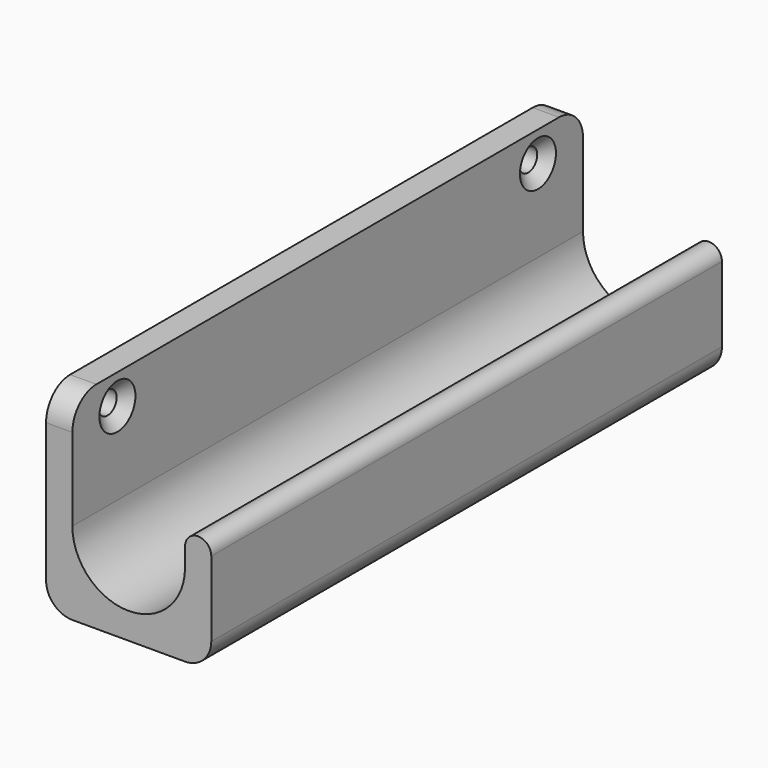
from build123d import *

# Parameters (mm, degrees)
F1_DEPTH  = 107.95
F3_R      = 1.5875
F2_R      = 1.905
F4_DEPTH  = 25.4
F5_SIZE2  = 1.4351924041
F5_SIZE   = 1.651
F7_DEPTH  = 107.95
F8_R      = 1.905
F9_DEPTH  = 25.4
F10_SIZE2 = 1.6559912355
F10_SIZE  = 1.905
F11_R     = 5.08


with BuildPart() as f1:
    # F0 (on Front) → F1 (new body)
    with BuildSketch(Plane.XZ):
        with BuildLine():
            Line((3.175, 0), (0, 0))
            Line((0, 0), (0, -28.575))
            ThreePointArc((0, -28.575), (0.9299359697, -30.8200640303), (3.175, -31.75))
            Line((3.175, -31.75), (22.225, -31.75))
            ThreePointArc((22.225, -31.75), (24.4700640303, -30.8200640303), (25.4, -28.575))
            Line((25.4, -28.575), (25.4, -15.875))
            ThreePointArc((25.4, -15.875), (23.8125, -14.2875), (22.225, -15.875))
            Line((22.225, -15.875), (22.225, -19.05))
            ThreePointArc((22.225, -19.05), (12.7, -28.575), (3.175, -19.05))
            Line((3.175, -19.05), (3.175, 0))
        make_face()
    extrude(amount=F1_DEPTH)

    # F3
    f3_edges = [f1.edges().sort_by_distance(p)[0] for p in [
        (1.5875, 0, 0),
        (1.5875, -107.95, 0),
    ]]
    fillet(f3_edges, radius=F3_R)

    # F2 (on face) → F4 (cut)
    with BuildSketch(Plane(origin=(0, 0, 0), x_dir=(0, -1, 0), z_dir=(-1, 0, 0))):
        with Locations((9.525, -5.08)):
            Circle(F2_R)
        with Locations((98.425, -5.08)):
            Circle(F2_R)
    extrude(amount=-F4_DEPTH, mode=Mode.SUBTRACT)

    # F5
    f5_edges = [f1.edges().sort_by_distance(p)[0] for p in [
        (3.175, -96.52, -5.08),
        (3.175, -7.62, -5.08),
    ]]
    chamfer(f5_edges, length=F5_SIZE, length2=F5_SIZE2)

    # F6 (on face) → F7 (join, through all)
    with BuildSketch(Plane.XZ.offset(107.95)):
        with BuildLine():
            Line((3.175, 0), (0, 0))
            Line((0, 0), (0, -28.575))
            ThreePointArc((0, -28.575), (0.9299359697, -30.8200640303), (3.175, -31.75))
            Line((3.175, -31.75), (22.225, -31.75))
            ThreePointArc((22.225, -31.75), (24.4700640303, -30.8200640303), (25.4, -28.575))
            Line((25.4, -28.575), (25.4, -15.875))
            ThreePointArc((25.4, -15.875), (23.8125, -14.2875), (22.225, -15.875))
            Line((22.225, -15.875), (22.225, -19.05))
            ThreePointArc((22.225, -19.05), (12.7, -28.575), (3.175, -19.05))
            Line((3.175, -19.05), (3.175, 0))
        make_face()
        with BuildLine():
            Line((0, -28.575), (0, 0))
            Line((0, 0), (-1.27, 0))
            Line((-1.27, 0), (-1.27, -28.575))
            ThreePointArc((-1.27, -28.575), (0.0319103576, -31.7180896424), (3.175, -33.02))
            Line((3.175, -33.02), (22.225, -33.02))
            ThreePointArc((22.225, -33.02), (25.3680896424, -31.7180896424), (26.67, -28.575))
            Line((26.67, -28.575), (26.67, -15.875))
            ThreePointArc((26.67, -15.875), (24.4475, -13.6525), (22.225, -15.875))
            ThreePointArc((22.225, -15.875), (23.8125, -14.2875), (25.4, -15.875))
            Line((25.4, -15.875), (25.4, -28.575))
            ThreePointArc((25.4, -28.575), (24.4700640303, -30.8200640303), (22.225, -31.75))
            Line((22.225, -31.75), (3.175, -31.75))
            ThreePointArc((3.175, -31.75), (0.9299359697, -30.8200640303), (0, -28.575))
        make_face()
    extrude(amount=-F7_DEPTH)

    # F8 (on face) → F9 (cut)
    with BuildSketch(Plane(origin=(-1.27, 0, 0), x_dir=(0, -1, 0), z_dir=(-1, 0, 0))):
        with Locations((9.525, -5.08)):
            Circle(F8_R)
        with Locations((98.425, -5.08)):
            Circle(F8_R)
    extrude(amount=-F9_DEPTH, mode=Mode.SUBTRACT)

    # F10
    f10_edges = [f1.edges().sort_by_distance(p)[0] for p in [
        (3.175, -96.52, -5.08),
        (3.175, -7.62, -5.08),
    ]]
    chamfer(f10_edges, length=F10_SIZE, length2=F10_SIZE2)

    # F11
    f11_edges = [f1.edges().sort_by_distance(p)[0] for p in [
        (0.9525, -107.95, 0),
        (0.9525, 0, 0),
    ]]
    fillet(f11_edges, radius=F11_R)


solid = f1.part
